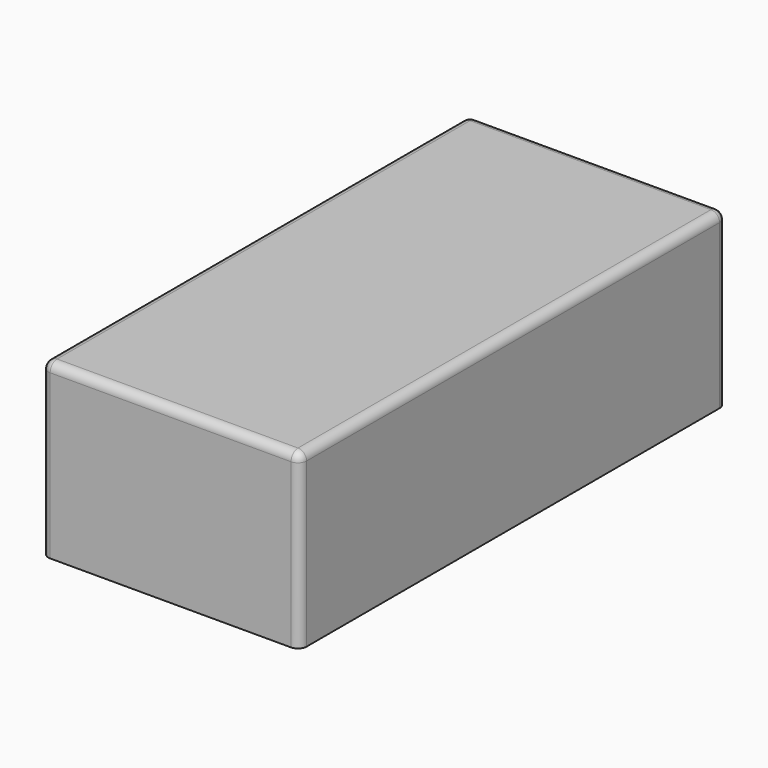
from build123d import *

# Parameters (mm, degrees)
F0_W     = 914.4
F0_H     = 1889.76
F1_DEPTH = 609.6
F3_R     = 30.48


# Not quite as in the source:
# - a feature of the source that left no trace in its solid (it failed there, or was rolled back) is left out


with BuildPart() as f1:
    # F0 (on Top) → F1 (new body)
    with BuildSketch(Plane.XY):
        with Locations((-13.0748171359, -203.4263992494)):
            Rectangle(F0_W, F0_H)
    extrude(amount=F1_DEPTH)

    # F3
    f3_edges = [f1.edges().sort_by_distance(p)[0] for p in [
        (-470.274817, -1148.306399, 304.8),
        (444.125183, -1148.306399, 304.8),
        (-13.074817, -1148.306399, 609.6),
        (444.125183, 741.453601, 304.8),
        (444.125183, -203.426399, 609.6),
        (-470.274817, 741.453601, 304.8),
        (-13.074817, 741.453601, 609.6),
        (-470.274817, -203.426399, 609.6),
    ]]
    fillet(f3_edges, radius=F3_R)


solid = f1.part
